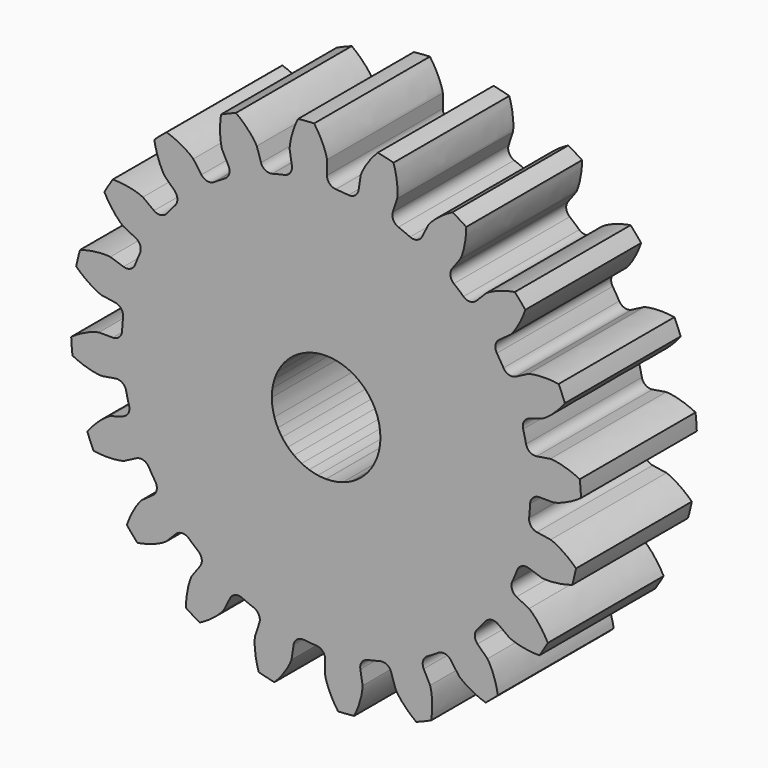
from build123d import *

# Parameters (mm, degrees)
F3_DEPTH        = 3.175
F3_COPIES_COUNT = 20
F4_R            = 0.2032


# Not quite as in the source:
# - a feature of the source that left no trace in its solid (it failed there, or was rolled back) is left out
# - a pattern or mirror of a feature is missing from the dataset's text; its kind, count and spacing are read off the source's solid


with BuildPart() as f3:
    # F2 (on Front) → F3 (new body)
    with BuildSketch(Plane.XZ):
        with BuildLine():
            add(Edge.make_bspline(
                [(-0.2623271276, 5.5922179347), (-0.1849689769, 5.4750736148), (-0.2062962503, 5.5111347034), (-0.1163695428, 5.3590826853), (-0.0738693263, 5.2704321119), (-0.034388462, 5.1765465004), (-0.009618674, 5.1074612872), (0.0141605918, 5.018472428), (0.0095740993, 5.0356364035), (0.0205723431, 4.9846737343)],
                knots=[0, 0, 0, 0, 0.1745368288, 0.3397849765, 0.4951362768, 0.6398645434, 0.7730772886, 0.8936346696, 1, 1, 1, 1], degree=3))
            ThreePointArc((-0.2623271276, 5.5922179347), (-0.4392428396, 5.5811094488), (-0.6157181757, 5.5644054561))
            add(Edge.make_bspline(
                [(-0.6157181757, 5.5644054561), (-0.6737985101, 5.4366018962), (-0.658375008, 5.4755553335), (-0.7234083924, 5.3113076917), (-0.7515173557, 5.2171000553), (-0.7758251996, 5.1181941637), (-0.789482722, 5.0460846555), (-0.799048301, 4.9544715001), (-0.7972033131, 4.9721416442), (-0.8000938325, 4.9200859055)],
                knots=[0, 0, 0, 0, 0.1745368288, 0.3397849765, 0.4951362768, 0.6398645434, 0.7730772886, 0.8936346696, 1, 1, 1, 1], degree=3))
            Line((-0.8000938325, 4.9200859055), (-0.719122101, 4.4221594638))
            ThreePointArc((-0.719122101, 4.4221594638), (-0.3515162836, 4.4664378672), (0.0184903645, 4.4802108238))
            Line((0.0184903645, 4.4802108238), (0.0205723431, 4.9846737343))
        make_face()
        with BuildLine():
            Line((0.0049138096, 1.1906148601), (0.0184903645, 4.4802108238))
            ThreePointArc((0.0184903645, 4.4802108238), (-0.3515162836, 4.4664378672), (-0.719122101, 4.4221594638))
            Line((-0.719122101, 4.4221594638), (-0.1911065111, 1.1751877263))
            ThreePointArc((-0.1911065111, 1.1751877263), (-0.0934153609, 1.1869547005), (0.0049138096, 1.1906148601))
        make_face()
        with BuildLine():
            ThreePointArc((4.4802489796, 0), (3.1745450348, 3.1614703448), (0.0184903645, 4.4802108238))
            Line((0.0184903645, 4.4802108238), (0.0049138096, 1.1906148601))
            ThreePointArc((0.0049138096, 1.1906148601), (0.8436345166, 0.8401599211), (1.190625, 0))
            ThreePointArc((1.190625, 0), (-0.7713791872, -0.9069520606), (-0.1911065111, 1.1751877263))
            Line((-0.1911065111, 1.1751877263), (-0.719122101, 4.4221594638))
            ThreePointArc((-0.719122101, 4.4221594638), (-2.9026526541, -3.4128050763), (4.4802489796, 0))
        make_face()
    extrude(amount=F3_DEPTH)

    # F3_copies: F3 ×20 about axis
    f3_copies_axis = Axis((0, 0, 0), (0, 1, 0))


with BuildPart() as f3_1:
    add(f3.part)
    for i in range(1, F3_COPIES_COUNT):
        add(f3.part.rotate(f3_copies_axis, i * 360 / F3_COPIES_COUNT))

    # F4
    f4_edges = [f3_1.edges().sort_by_distance(p)[0] for p in [
        (-0.719122, -1.5875, 4.422159),
        (-1.366876, -1.5875, 4.266648),
        (-2.050448, -1.5875, 3.983503),
        (-2.618443, -1.5875, 3.635435),
        (-3.181062, -1.5875, 3.154913),
        (-3.613698, -1.5875, 2.648361),
        (-4.000292, -1.5875, 2.017498),
        (-4.25522, -1.5875, 1.402047),
        (-4.427945, -1.5875, 0.682597),
        (-4.480211, -1.5875, 0.01849),
        (-4.422159, -1.5875, -0.719122),
        (-4.266648, -1.5875, -1.366876),
        (-3.983503, -1.5875, -2.050448),
        (-3.635435, -1.5875, -2.618443),
        (-3.154913, -1.5875, -3.181062),
        (-2.648361, -1.5875, -3.613698),
        (-2.017498, -1.5875, -4.000292),
        (-1.402047, -1.5875, -4.25522),
        (-0.682597, -1.5875, -4.427945),
        (-0.01849, -1.5875, -4.480211),
        (0.719122, -1.5875, -4.422159),
        (1.366876, -1.5875, -4.266648),
        (2.050448, -1.5875, -3.983503),
        (2.618443, -1.5875, -3.635435),
        (3.181062, -1.5875, -3.154913),
        (3.613698, -1.5875, -2.648361),
        (4.000292, -1.5875, -2.017498),
        (4.25522, -1.5875, -1.402047),
        (4.427945, -1.5875, -0.682597),
        (4.480211, -1.5875, -0.01849),
        (4.422159, -1.5875, 0.719122),
        (4.266648, -1.5875, 1.366876),
        (3.983503, -1.5875, 2.050448),
        (3.635435, -1.5875, 2.618443),
        (3.154913, -1.5875, 3.181062),
        (2.648361, -1.5875, 3.613698),
        (2.017498, -1.5875, 4.000292),
        (1.402047, -1.5875, 4.25522),
        (0.682597, -1.5875, 4.427945),
        (0.01849, -1.5875, 4.480211),
    ]]
    fillet(f4_edges, radius=F4_R)


solid = f3_1.part
